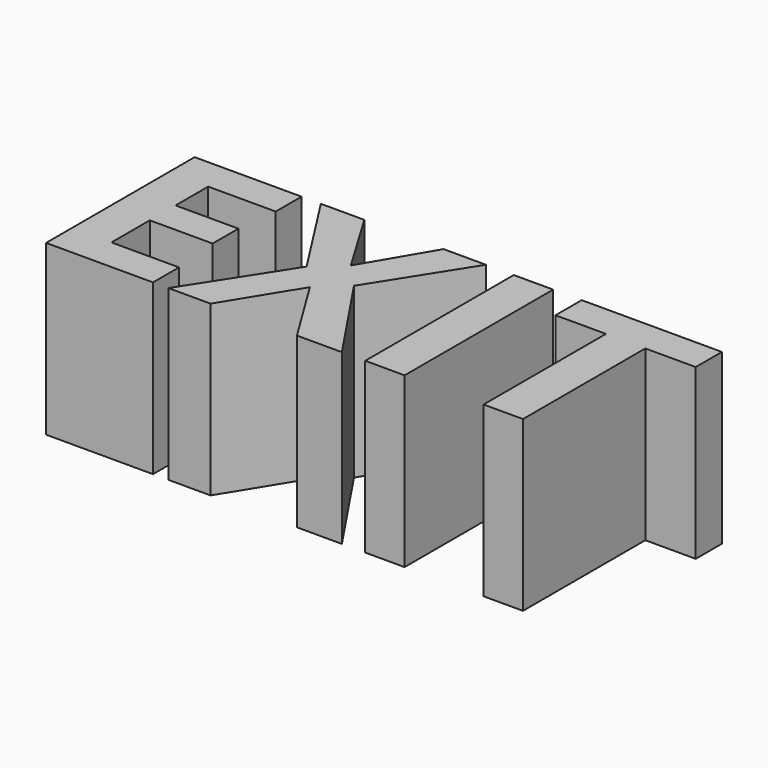
from build123d import *

# Parameters (mm, degrees)
F0_TEXT_SIZE = 39.1256788539
F1_DEPTH     = 25.4


# Not quite as in the source:
# - Text() gives the source's letters only with a copy of the font that has no kerning and outlines rounded to 1/6400 em; it was checked with that copy


with BuildPart() as f1:
    # F0 (on Top) → F1 (new body)
    with BuildSketch(Plane.XY):
        with Locations((-44.2886576056, 4.3562613428)):
            Text('EXIT', F0_TEXT_SIZE, font='Open Sans', font_style=FontStyle.BOLD, text_align=(TextAlign.LEFT, TextAlign.BOTTOM))
    extrude(amount=F1_DEPTH)


solid = f1.part
